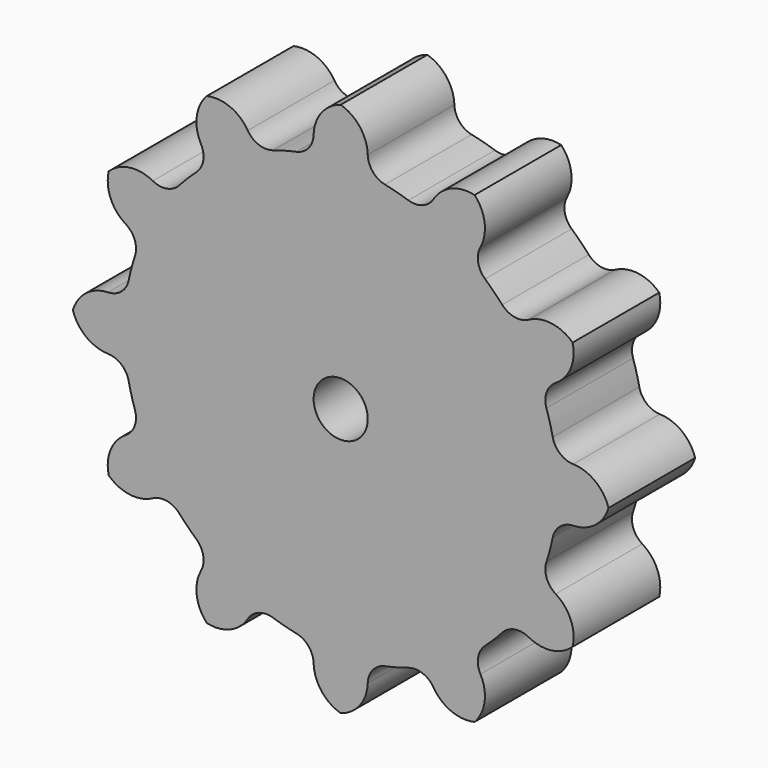
from build123d import *

# Parameters (mm, degrees)
F1_DEPTH    = 25.4
F3_DEPTH    = 25.4
F4_R        = 6.35
F5_DEPTH    = 25.4
F6_T1_DEPTH = 69.85
F7_R        = 5.08


# Not quite as in the source:
# - a fillet or chamfer that OpenCascade refuses, or shapes differently, is made with other operations: its cross-section is extruded or revolved along the edge and cut away or added
# - a feature names something its author has since deleted; it is built from what else it names


with BuildPart() as f1:
    # F0 (on Front) → F1 (new body)
    with BuildSketch(Plane.XZ):
        with BuildLine():
            ThreePointArc((19.7015199239, 46.8240334945), (25.4, 43.9940905122), (30.7000425519, 40.4740334945))
            Line((30.7000425519, 40.4740334945), (37.0901124422, 51.5419592083))
            Line((37.0901124422, 51.5419592083), (26.0915898141, 57.8919592083))
            Line((26.0915898141, 57.8919592083), (19.7015199239, 46.8240334945))
        make_face()
        with BuildLine():
            ThreePointArc((-6.35, 50.4015624758), (0, 50.8), (6.35, 50.4015624758))
            Line((6.35, 50.4015624758), (6.35, 63.1817022563))
            Line((6.35, 63.1817022563), (-6.35, 63.1817022563))
            Line((-6.35, 63.1817022563), (-6.35, 50.4015624758))
        make_face()
        with BuildLine():
            Line((-26.0915898141, -57.8919592083), (-19.7015199239, -46.8240334945))
            ThreePointArc((-19.7015199239, -46.8240334945), (-25.4, -43.9940905122), (-30.7000425519, -40.4740334945))
            Line((-30.7000425519, -40.4740334945), (-37.0901124422, -51.5419592083))
            Line((-37.0901124422, -51.5419592083), (-26.0915898141, -57.8919592083))
        make_face()
        with BuildLine():
            Line((6.35, -63.1817022563), (6.35, -50.4015624758))
            ThreePointArc((6.35, -50.4015624758), (0, -50.8), (-6.35, -50.4015624758))
            Line((-6.35, -50.4015624758), (-6.35, -63.1817022563))
            Line((-6.35, -63.1817022563), (6.35, -63.1817022563))
        make_face()
        with BuildLine():
            Line((30.7000425519, 40.4740334945), (17.3485226281, 17.3485226281))
            Line((17.3485226281, 17.3485226281), (40.4740334945, 30.7000425519))
            ThreePointArc((40.4740334945, 30.7000425519), (35.9210244843, 35.9210244843), (30.7000425519, 40.4740334945))
        make_face()
        with BuildLine():
            Line((6.35, 50.4015624758), (6.35, 23.6985226281))
            Line((6.35, 23.6985226281), (19.7015199239, 46.8240334945))
            ThreePointArc((19.7015199239, 46.8240334945), (13.1480074912, 49.0690319755), (6.35, 50.4015624758))
        make_face()
        with BuildLine():
            Line((-46.8240334945, -19.7015199239), (-6.35, 3.6661742094))
            Line((-6.35, 3.6661742094), (-6.35, 50.4015624758))
            ThreePointArc((-6.35, 50.4015624758), (-43.9940905122, 25.4), (-46.8240334945, -19.7015199239))
        make_face()
        with BuildLine():
            Line((-6.35, -50.4015624758), (-6.35, -23.6985226281))
            Line((-6.35, -23.6985226281), (-19.7015199239, -46.8240334945))
            ThreePointArc((-19.7015199239, -46.8240334945), (-13.1480074912, -49.0690319755), (-6.35, -50.4015624758))
        make_face()
        with BuildLine():
            Line((-30.7000425519, -40.4740334945), (-6.35, 1.7014773719))
            Line((-6.35, 1.7014773719), (-6.35, 3.6661742094))
            Line((-6.35, 3.6661742094), (-46.8240334945, -19.7015199239))
            ThreePointArc((-46.8240334945, -19.7015199239), (-40.1294146696, -31.1491585485), (-30.7000425519, -40.4740334945))
        make_face()
        with BuildLine():
            Line((17.3485226281, 17.3485226281), (6.35, -1.7014773719))
            Line((6.35, -1.7014773719), (6.35, -50.4015624758))
            ThreePointArc((6.35, -50.4015624758), (38.1, -33.6010416505), (50.8, 0))
            ThreePointArc((50.8, 0), (48.149355663, 16.1950470589), (40.4740334945, 30.7000425519))
            Line((40.4740334945, 30.7000425519), (17.3485226281, 17.3485226281))
        make_face()
        with BuildLine():
            Line((6.35, 23.6985226281), (6.35, 10.9985226281))
            Line((6.35, 10.9985226281), (17.3485226281, 17.3485226281))
            Line((17.3485226281, 17.3485226281), (30.7000425519, 40.4740334945))
            ThreePointArc((30.7000425519, 40.4740334945), (25.4, 43.9940905122), (19.7015199239, 46.8240334945))
            Line((19.7015199239, 46.8240334945), (6.35, 23.6985226281))
        make_face()
        with BuildLine():
            Line((-6.35, 3.6661742094), (-4.6485226281, 4.6485226281))
            Line((-4.6485226281, 4.6485226281), (6.35, 23.6985226281))
            Line((6.35, 23.6985226281), (6.35, 50.4015624758))
            ThreePointArc((6.35, 50.4015624758), (0, 50.8), (-6.35, 50.4015624758))
            Line((-6.35, 50.4015624758), (-6.35, 3.6661742094))
        make_face()
        with BuildLine():
            Line((-6.35, -23.6985226281), (-6.35, 1.31e-08))
            Line((-6.35, 1.31e-08), (-6.35, 1.7014773719))
            Line((-6.35, 1.7014773719), (-30.7000425519, -40.4740334945))
            ThreePointArc((-30.7000425519, -40.4740334945), (-25.4, -43.9940905122), (-19.7015199239, -46.8240334945))
            Line((-19.7015199239, -46.8240334945), (-6.35, -23.6985226281))
        make_face()
        with BuildLine():
            Line((6.35, -1.7014773719), (5.4992613469, -3.1749999431))
            Line((5.4992613469, -3.1749999431), (-6.35, -23.6985226281))
            Line((-6.35, -23.6985226281), (-6.35, -50.4015624758))
            ThreePointArc((-6.35, -50.4015624758), (0, -50.8), (6.35, -50.4015624758))
            Line((6.35, -50.4015624758), (6.35, -1.7014773719))
        make_face()
        Polygon((-4.6485226281, 4.6485226281), (-3.1750000958, 5.4992612587), (6.35, 10.9985226281), (6.35, 23.6985226281), align=None)
        with BuildLine():
            ThreePointArc((5.4992613469, -3.1749999431), (6.1336290054, -1.6435009047), (6.35, 0))
            ThreePointArc((6.35, 0), (3.1749999521, 5.4992613417), (-3.1750000958, 5.4992612587))
            ThreePointArc((-3.1750000958, 5.4992612587), (-4.490128147, 4.490127974), (-5.499261381, 3.1749998839))
            ThreePointArc((-5.499261381, 3.1749998839), (-6.1336290126, 1.643500878), (-6.35, 1.31e-08))
            ThreePointArc((-6.35, 1.31e-08), (-1.643500911, -6.1336290037), (5.4992613469, -3.1749999431))
        make_face()
        Polygon((6.35, 10.9985226281), (6.35, 0), (6.35, -1.7014773719), (17.3485226281, 17.3485226281), align=None)
        with BuildLine():
            ThreePointArc((-3.1750000958, 5.4992612587), (3.1749999521, 5.4992613417), (6.35, 0))
            Line((6.35, 0), (6.35, 10.9985226281))
            Line((6.35, 10.9985226281), (-3.1750000958, 5.4992612587))
        make_face()
        with BuildLine():
            Line((-6.35, -23.6985226281), (5.4992613469, -3.1749999431))
            ThreePointArc((5.4992613469, -3.1749999431), (-1.643500911, -6.1336290037), (-6.35, 1.31e-08))
            Line((-6.35, 1.31e-08), (-6.35, -23.6985226281))
        make_face()
        Polygon((-6.35, 1.7014773719), (-5.499261381, 3.1749998839), (-4.6485226281, 4.6485226281), (-6.35, 3.6661742094), align=None)
        with BuildLine():
            Line((6.35, -1.7014773719), (6.35, 0))
            ThreePointArc((6.35, 0), (6.1336290054, -1.6435009047), (5.4992613469, -3.1749999431))
            Line((5.4992613469, -3.1749999431), (6.35, -1.7014773719))
        make_face()
        with BuildLine():
            ThreePointArc((-5.499261381, 3.1749998839), (-4.490128147, 4.490127974), (-3.1750000958, 5.4992612587))
            Line((-3.1750000958, 5.4992612587), (-4.6485226281, 4.6485226281))
            Line((-4.6485226281, 4.6485226281), (-5.499261381, 3.1749998839))
        make_face()
        with BuildLine():
            ThreePointArc((-6.35, 1.31e-08), (-6.1336290126, 1.643500878), (-5.499261381, 3.1749998839))
            Line((-5.499261381, 3.1749998839), (-6.35, 1.7014773719))
            Line((-6.35, 1.7014773719), (-6.35, 1.31e-08))
        make_face()
    extrude(amount=F1_DEPTH)

    # F2 (on Front) → F3 (join)
    with BuildSketch(Plane.XZ):
        with BuildLine():
            ThreePointArc((40.4740334945, 30.7000425519), (43.9940905122, 25.4), (46.8240334945, 19.7015199239))
            Line((46.8240334945, 19.7015199239), (57.8919592083, 26.0915898141))
            Line((57.8919592083, 26.0915898141), (51.5419592083, 37.0901124422))
            Line((51.5419592083, 37.0901124422), (40.4740334945, 30.7000425519))
        make_face()
        with BuildLine():
            ThreePointArc((-30.7000425519, 40.4740334945), (-25.4, 43.9940905122), (-19.7015199239, 46.8240334945))
            Line((-19.7015199239, 46.8240334945), (-26.0915898141, 57.8919592083))
            Line((-26.0915898141, 57.8919592083), (-37.0901124422, 51.5419592083))
            Line((-37.0901124422, 51.5419592083), (-30.7000425519, 40.4740334945))
        make_face()
        with BuildLine():
            ThreePointArc((-46.8240334945, 19.7015199239), (-43.9940905122, 25.4), (-40.4740334945, 30.7000425519))
            Line((-40.4740334945, 30.7000425519), (-51.5419592083, 37.0901124422))
            Line((-51.5419592083, 37.0901124422), (-57.8919592083, 26.0915898141))
            Line((-57.8919592083, 26.0915898141), (-46.8240334945, 19.7015199239))
        make_face()
        with BuildLine():
            Line((-63.1817022563, -6.35), (-50.4015624758, -6.35))
            ThreePointArc((-50.4015624758, -6.35), (-50.8, 0), (-50.4015624758, 6.35))
            Line((-50.4015624758, 6.35), (-63.1817022563, 6.35))
            Line((-63.1817022563, 6.35), (-63.1817022563, -6.35))
        make_face()
        with BuildLine():
            Line((-51.5419592083, -37.0901124422), (-40.4740334945, -30.7000425519))
            ThreePointArc((-40.4740334945, -30.7000425519), (-43.9940905122, -25.4), (-46.8240334945, -19.7015199239))
            Line((-46.8240334945, -19.7015199239), (-57.8919592083, -26.0915898141))
            Line((-57.8919592083, -26.0915898141), (-51.5419592083, -37.0901124422))
        make_face()
        with BuildLine():
            Line((37.0901124422, -51.5419592083), (30.7000425519, -40.4740334945))
            ThreePointArc((30.7000425519, -40.4740334945), (25.4, -43.9940905122), (19.7015199239, -46.8240334945))
            Line((19.7015199239, -46.8240334945), (26.0915898141, -57.8919592083))
            Line((26.0915898141, -57.8919592083), (37.0901124422, -51.5419592083))
        make_face()
        with BuildLine():
            Line((57.8919592083, -26.0915898141), (46.8240334945, -19.7015199239))
            ThreePointArc((46.8240334945, -19.7015199239), (43.9940905122, -25.4), (40.4740334945, -30.7000425519))
            Line((40.4740334945, -30.7000425519), (51.5419592083, -37.0901124422))
            Line((51.5419592083, -37.0901124422), (57.8919592083, -26.0915898141))
        make_face()
        with BuildLine():
            Line((63.1817022563, 6.35), (50.4015624758, 6.35))
            ThreePointArc((50.4015624758, 6.35), (50.7002927692, 3.1812439572), (50.8, 0))
            ThreePointArc((50.8, 0), (50.7002927692, -3.1812439572), (50.4015624758, -6.35))
            Line((50.4015624758, -6.35), (63.1817022563, -6.35))
            Line((63.1817022563, -6.35), (63.1817022563, 6.35))
        make_face()
        with BuildLine():
            Line((46.8240334945, 19.7015199239), (23.6985226281, 6.35))
            Line((23.6985226281, 6.35), (50.4015624758, 6.35))
            ThreePointArc((50.4015624758, 6.35), (49.0690319755, 13.1480074912), (46.8240334945, 19.7015199239))
        make_face()
        with BuildLine():
            Line((-19.7015199239, 46.8240334945), (2.324261314, 8.674261314))
            Line((2.324261314, 8.674261314), (40.4740334945, 30.7000425519))
            ThreePointArc((40.4740334945, 30.7000425519), (13.1480074912, 49.0690319755), (-19.7015199239, 46.8240334945))
        make_face()
        with BuildLine():
            Line((-40.4740334945, 30.7000425519), (-17.3485226281, 17.3485226281))
            Line((-17.3485226281, 17.3485226281), (-30.7000425519, 40.4740334945))
            ThreePointArc((-30.7000425519, 40.4740334945), (-35.9210244843, 35.9210244843), (-40.4740334945, 30.7000425519))
        make_face()
        with BuildLine():
            Line((-50.4015624758, 6.35), (-23.6985226281, 6.35))
            Line((-23.6985226281, 6.35), (-46.8240334945, 19.7015199239))
            ThreePointArc((-46.8240334945, 19.7015199239), (-49.0690319755, 13.1480074912), (-50.4015624758, 6.35))
        make_face()
        with BuildLine():
            Line((-46.8240334945, -19.7015199239), (-23.6985226281, -6.35))
            Line((-23.6985226281, -6.35), (-50.4015624758, -6.35))
            ThreePointArc((-50.4015624758, -6.35), (-49.0690319755, -13.1480074912), (-46.8240334945, -19.7015199239))
        make_face()
        with BuildLine():
            Line((19.7015199239, -46.8240334945), (-2.324261314, -8.674261314))
            Line((-2.324261314, -8.674261314), (-40.4740334945, -30.7000425519))
            ThreePointArc((-40.4740334945, -30.7000425519), (-13.1480074912, -49.0690319755), (19.7015199239, -46.8240334945))
        make_face()
        with BuildLine():
            Line((40.4740334945, -30.7000425519), (17.3485226281, -17.3485226281))
            Line((17.3485226281, -17.3485226281), (30.7000425519, -40.4740334945))
            ThreePointArc((30.7000425519, -40.4740334945), (35.9210244843, -35.9210244843), (40.4740334945, -30.7000425519))
        make_face()
        with BuildLine():
            Line((50.4015624758, -6.35), (23.6985226281, -6.35))
            Line((23.6985226281, -6.35), (46.8240334945, -19.7015199239))
            ThreePointArc((46.8240334945, -19.7015199239), (49.0690319755, -13.1480074912), (50.4015624758, -6.35))
        make_face()
        with BuildLine():
            Line((2.324261314, 8.674261314), (3.6661742094, 6.35))
            Line((3.6661742094, 6.35), (23.6985226281, 6.35))
            Line((23.6985226281, 6.35), (46.8240334945, 19.7015199239))
            ThreePointArc((46.8240334945, 19.7015199239), (43.9940905122, 25.4), (40.4740334945, 30.7000425519))
            Line((40.4740334945, 30.7000425519), (2.324261314, 8.674261314))
        make_face()
        with BuildLine():
            Line((-17.3485226281, 17.3485226281), (0, 7.3323484187))
            Line((0, 7.3323484187), (2.324261314, 8.674261314))
            Line((2.324261314, 8.674261314), (-19.7015199239, 46.8240334945))
            ThreePointArc((-19.7015199239, 46.8240334945), (-25.4, 43.9940905122), (-30.7000425519, 40.4740334945))
            Line((-30.7000425519, 40.4740334945), (-17.3485226281, 17.3485226281))
        make_face()
        with BuildLine():
            Line((-23.6985226281, 6.35), (-10.9985226281, 6.35))
            Line((-10.9985226281, 6.35), (-17.3485226281, 17.3485226281))
            Line((-17.3485226281, 17.3485226281), (-40.4740334945, 30.7000425519))
            ThreePointArc((-40.4740334945, 30.7000425519), (-43.9940905122, 25.4), (-46.8240334945, 19.7015199239))
            Line((-46.8240334945, 19.7015199239), (-23.6985226281, 6.35))
        make_face()
        with BuildLine():
            Line((-23.6985226281, -6.35), (-12.7, 0))
            Line((-12.7, 0), (-23.6985226281, 6.35))
            Line((-23.6985226281, 6.35), (-50.4015624758, 6.35))
            ThreePointArc((-50.4015624758, 6.35), (-50.8, 0), (-50.4015624758, -6.35))
            Line((-50.4015624758, -6.35), (-23.6985226281, -6.35))
        make_face()
        with BuildLine():
            Line((-2.324261314, -8.674261314), (-3.6661742094, -6.35))
            Line((-3.6661742094, -6.35), (-23.6985226281, -6.35))
            Line((-23.6985226281, -6.35), (-46.8240334945, -19.7015199239))
            ThreePointArc((-46.8240334945, -19.7015199239), (-43.9940905122, -25.4), (-40.4740334945, -30.7000425519))
            Line((-40.4740334945, -30.7000425519), (-2.324261314, -8.674261314))
        make_face()
        with BuildLine():
            Line((17.3485226281, -17.3485226281), (0, -7.3323484187))
            Line((0, -7.3323484187), (-2.324261314, -8.674261314))
            Line((-2.324261314, -8.674261314), (19.7015199239, -46.8240334945))
            ThreePointArc((19.7015199239, -46.8240334945), (25.4, -43.9940905122), (30.7000425519, -40.4740334945))
            Line((30.7000425519, -40.4740334945), (17.3485226281, -17.3485226281))
        make_face()
        with BuildLine():
            Line((23.6985226281, -6.35), (10.9985226281, -6.35))
            Line((10.9985226281, -6.35), (17.3485226281, -17.3485226281))
            Line((17.3485226281, -17.3485226281), (40.4740334945, -30.7000425519))
            ThreePointArc((40.4740334945, -30.7000425519), (43.9940905122, -25.4), (46.8240334945, -19.7015199239))
            Line((46.8240334945, -19.7015199239), (23.6985226281, -6.35))
        make_face()
        with BuildLine():
            Line((23.6985226281, 6.35), (12.7, 0))
            Line((12.7, 0), (23.6985226281, -6.35))
            Line((23.6985226281, -6.35), (50.4015624758, -6.35))
            ThreePointArc((50.4015624758, -6.35), (50.7002927692, -3.1812439572), (50.8, 0))
            ThreePointArc((50.8, 0), (50.7002927692, 3.1812439572), (50.4015624758, 6.35))
            Line((50.4015624758, 6.35), (23.6985226281, 6.35))
        make_face()
        Polygon((-12.7, 0), (-8.674261314, 2.324261314), (-10.9985226281, 6.35), (-23.6985226281, 6.35), align=None)
        with BuildLine():
            ThreePointArc((-5.4992614049, -3.1749998425), (-6.1336289764, 1.643501013), (-3.1750000201, 5.4992613024))
            Line((-3.1750000201, 5.4992613024), (-8.674261314, 2.324261314))
            Line((-8.674261314, 2.324261314), (-5.4992614049, -3.1749998425))
        make_face()
        Polygon((3.6661742094, 6.35), (4.6485226281, 4.6485226281), (12.7, 0), (23.6985226281, 6.35), align=None)
        Polygon((8.674261314, -2.324261314), (3.1750001359, -5.4992612355), (1.7014773719, -6.35), (10.9985226281, -6.35), align=None)
        Polygon((-3.6661742094, -6.35), (-4.6485226281, -4.6485226281), (-12.7, 0), (-23.6985226281, -6.35), align=None)
        Polygon((-10.9985226281, 6.35), (-1.7014773719, 6.35), (0, 7.3323484187), (-17.3485226281, 17.3485226281), align=None)
        Polygon((-4.6485226281, -4.6485226281), (-5.4992614049, -3.1749998425), (-8.674261314, 2.324261314), (-12.7, 0), align=None)
        Polygon((10.9985226281, -6.35), (1.7014773719, -6.35), (0, -7.3323484187), (17.3485226281, -17.3485226281), align=None)
        Polygon((4.6485226281, 4.6485226281), (5.4992613044, 3.1750000167), (8.674261314, -2.324261314), (12.7, 0), align=None)
        Polygon((0, -7.3323484187), (-1.7014773719, -6.35), (-3.6661742094, -6.35), (-2.324261314, -8.674261314), align=None)
        with BuildLine():
            ThreePointArc((5.4992613044, 3.1750000167), (6.1336289944, 1.6435009457), (6.35, 0))
            ThreePointArc((6.35, 0), (5.4992613533, -3.174999932), (3.1750001359, -5.4992612355))
            Line((3.1750001359, -5.4992612355), (8.674261314, -2.324261314))
            Line((8.674261314, -2.324261314), (5.4992613044, 3.1750000167))
        make_face()
        Polygon((-8.674261314, 2.324261314), (-3.1750000201, 5.4992613024), (-1.7014773719, 6.35), (-10.9985226281, 6.35), align=None)
        Polygon((12.7, 0), (8.674261314, -2.324261314), (10.9985226281, -6.35), (23.6985226281, -6.35), align=None)
        Polygon((1.7014773719, -6.35), (3.51e-08, -6.35), (-1.7014773719, -6.35), (0, -7.3323484187), align=None)
        Polygon((1.7014773719, 6.35), (3.1750001989, 5.4992611992), (4.6485226281, 4.6485226281), (3.6661742094, 6.35), align=None)
        Polygon((0, 7.3323484187), (1.7014773719, 6.35), (3.6661742094, 6.35), (2.324261314, 8.674261314), align=None)
        Polygon((-1.7014773719, -6.35), (-3.174999941, -5.4992613481), (-4.6485226281, -4.6485226281), (-3.6661742094, -6.35), align=None)
        with BuildLine():
            ThreePointArc((3.1750001359, -5.4992612355), (5.4992613533, -3.174999932), (6.35, 0))
            ThreePointArc((6.35, 0), (6.1336289944, 1.6435009457), (5.4992613044, 3.1750000167))
            ThreePointArc((5.4992613044, 3.1750000167), (4.4901281349, 4.4901279862), (3.1750001989, 5.4992611992))
            ThreePointArc((3.1750001989, 5.4992611992), (1.6435010473, 6.1336289672), (0, 6.35))
            ThreePointArc((0, 6.35), (-1.6435009476, 6.1336289939), (-3.1750000201, 5.4992613024))
            ThreePointArc((-3.1750000201, 5.4992613024), (-6.1336289764, 1.643501013), (-5.4992614049, -3.1749998425))
            ThreePointArc((-5.4992614049, -3.1749998425), (-4.4901281007, -4.4901280203), (-3.174999941, -5.4992613481))
            ThreePointArc((-3.174999941, -5.4992613481), (-1.6435008865, -6.1336290103), (3.51e-08, -6.35))
            ThreePointArc((3.51e-08, -6.35), (1.6435010292, -6.1336289721), (3.1750001359, -5.4992612355))
        make_face()
        with BuildLine():
            ThreePointArc((-3.1750000201, 5.4992613024), (-1.6435009476, 6.1336289939), (0, 6.35))
            Line((0, 6.35), (-1.7014773719, 6.35))
            Line((-1.7014773719, 6.35), (-3.1750000201, 5.4992613024))
        make_face()
        with BuildLine():
            Line((1.7014773719, -6.35), (3.1750001359, -5.4992612355))
            ThreePointArc((3.1750001359, -5.4992612355), (1.6435010292, -6.1336289721), (3.51e-08, -6.35))
            Line((3.51e-08, -6.35), (1.7014773719, -6.35))
        make_face()
        Polygon((-1.7014773719, 6.35), (0, 6.35), (1.7014773719, 6.35), (0, 7.3323484187), align=None)
        with BuildLine():
            ThreePointArc((0, 6.35), (1.6435010473, 6.1336289672), (3.1750001989, 5.4992611992))
            Line((3.1750001989, 5.4992611992), (1.7014773719, 6.35))
            Line((1.7014773719, 6.35), (0, 6.35))
        make_face()
        with BuildLine():
            Line((-1.7014773719, -6.35), (3.51e-08, -6.35))
            ThreePointArc((3.51e-08, -6.35), (-1.6435008865, -6.1336290103), (-3.174999941, -5.4992613481))
            Line((-3.174999941, -5.4992613481), (-1.7014773719, -6.35))
        make_face()
        with BuildLine():
            Line((-4.6485226281, -4.6485226281), (-3.174999941, -5.4992613481))
            ThreePointArc((-3.174999941, -5.4992613481), (-4.4901281007, -4.4901280203), (-5.4992614049, -3.1749998425))
            Line((-5.4992614049, -3.1749998425), (-4.6485226281, -4.6485226281))
        make_face()
        with BuildLine():
            ThreePointArc((3.1750001989, 5.4992611992), (4.4901281349, 4.4901279862), (5.4992613044, 3.1750000167))
            Line((5.4992613044, 3.1750000167), (4.6485226281, 4.6485226281))
            Line((4.6485226281, 4.6485226281), (3.1750001989, 5.4992611992))
        make_face()
    extrude(amount=F3_DEPTH)

    # F4 (on face) → F5 (cut)
    with BuildSketch(Plane.XZ.offset(25.4)):
        Circle(F4_R)
    extrude(amount=-F5_DEPTH, mode=Mode.SUBTRACT)

    # F6: fillet of radius 8.89 on 24 edges, made by hand

    # F6_s2 → F6_t1 (cut)
    with BuildSketch(Plane.XZ.offset(-22.225)):
        with BuildLine():
            ThreePointArc((2.54, 63.1817022563), (-3.7461792847, 60.577881541), (-6.35, 54.2917022563))
            Line((-6.35, 54.2917022563), (-6.35, 63.1817022563))
            Line((-6.35, 63.1817022563), (2.54, 63.1817022563))
        make_face()
        with BuildLine():
            ThreePointArc((6.35, 54.2917022563), (3.7461792847, 60.577881541), (-2.54, 63.1817022563))
            Line((-2.54, 63.1817022563), (6.35, 63.1817022563))
            Line((6.35, 63.1817022563), (6.35, 54.2917022563))
        make_face()
        with BuildLine():
            ThreePointArc((33.7905556537, 53.4469592083), (27.0446543428, 54.3350739643), (21.6465898141, 50.1929933686))
            Line((21.6465898141, 50.1929933686), (26.0915898141, 57.8919592083))
            Line((26.0915898141, 57.8919592083), (33.7905556537, 53.4469592083))
        make_face()
        with BuildLine():
            ThreePointArc((32.6451124422, 43.8429933686), (33.5332271982, 50.5888946796), (29.3911466025, 55.9869592083))
            Line((29.3911466025, 55.9869592083), (37.0901124422, 51.5419592083))
            Line((37.0901124422, 51.5419592083), (32.6451124422, 43.8429933686))
        make_face()
        with BuildLine():
            ThreePointArc((43.8429933686, 32.6451124422), (50.5888946796, 33.5332271982), (55.9869592083, 29.3911466025))
            Line((55.9869592083, 29.3911466025), (51.5419592083, 37.0901124422))
            Line((51.5419592083, 37.0901124422), (43.8429933686, 32.6451124422))
        make_face()
        with BuildLine():
            ThreePointArc((53.4469592083, 33.7905556537), (54.3350739643, 27.0446543428), (50.1929933686, 21.6465898141))
            Line((50.1929933686, 21.6465898141), (57.8919592083, 26.0915898141))
            Line((57.8919592083, 26.0915898141), (53.4469592083, 33.7905556537))
        make_face()
        with BuildLine():
            ThreePointArc((-21.6465898141, 50.1929933686), (-27.0446543428, 54.3350739643), (-33.7905556537, 53.4469592083))
            Line((-33.7905556537, 53.4469592083), (-26.0915898141, 57.8919592083))
            Line((-26.0915898141, 57.8919592083), (-21.6465898141, 50.1929933686))
        make_face()
        with BuildLine():
            ThreePointArc((-29.3911466025, 55.9869592083), (-33.5332271982, 50.5888946796), (-32.6451124422, 43.8429933686))
            Line((-32.6451124422, 43.8429933686), (-37.0901124422, 51.5419592083))
            Line((-37.0901124422, 51.5419592083), (-29.3911466025, 55.9869592083))
        make_face()
        with BuildLine():
            ThreePointArc((-43.8429933686, 32.6451124422), (-50.5888946796, 33.5332271982), (-55.9869592083, 29.3911466025))
            Line((-55.9869592083, 29.3911466025), (-51.5419592083, 37.0901124422))
            Line((-51.5419592083, 37.0901124422), (-43.8429933686, 32.6451124422))
        make_face()
        with BuildLine():
            ThreePointArc((-53.4469592083, 33.7905556537), (-54.3350739643, 27.0446543428), (-50.1929933686, 21.6465898141))
            Line((-50.1929933686, 21.6465898141), (-57.8919592083, 26.0915898141))
            Line((-57.8919592083, 26.0915898141), (-53.4469592083, 33.7905556537))
        make_face()
        with BuildLine():
            ThreePointArc((-54.2917022563, 6.35), (-60.577881541, 3.7461792847), (-63.1817022563, -2.54))
            Line((-63.1817022563, -2.54), (-63.1817022563, 6.35))
            Line((-63.1817022563, 6.35), (-54.2917022563, 6.35))
        make_face()
        with BuildLine():
            ThreePointArc((-63.1817022563, 2.54), (-60.577881541, -3.7461792847), (-54.2917022563, -6.35))
            Line((-54.2917022563, -6.35), (-63.1817022563, -6.35))
            Line((-63.1817022563, -6.35), (-63.1817022563, 2.54))
        make_face()
        with BuildLine():
            ThreePointArc((-55.9869592083, -29.3911466025), (-50.5888946796, -33.5332271982), (-43.8429933686, -32.6451124422))
            Line((-43.8429933686, -32.6451124422), (-51.5419592083, -37.0901124422))
            Line((-51.5419592083, -37.0901124422), (-55.9869592083, -29.3911466025))
        make_face()
        with BuildLine():
            ThreePointArc((-50.1929933686, -21.6465898141), (-54.3350739643, -27.0446543428), (-53.4469592083, -33.7905556537))
            Line((-53.4469592083, -33.7905556537), (-57.8919592083, -26.0915898141))
            Line((-57.8919592083, -26.0915898141), (-50.1929933686, -21.6465898141))
        make_face()
        with BuildLine():
            ThreePointArc((-32.6451124422, -43.8429933686), (-33.5332271982, -50.5888946796), (-29.3911466025, -55.9869592083))
            Line((-29.3911466025, -55.9869592083), (-37.0901124422, -51.5419592083))
            Line((-37.0901124422, -51.5419592083), (-32.6451124422, -43.8429933686))
        make_face()
        with BuildLine():
            ThreePointArc((-33.7905556537, -53.4469592083), (-27.0446543428, -54.3350739643), (-21.6465898141, -50.1929933686))
            Line((-21.6465898141, -50.1929933686), (-26.0915898141, -57.8919592083))
            Line((-26.0915898141, -57.8919592083), (-33.7905556537, -53.4469592083))
        make_face()
        with BuildLine():
            ThreePointArc((2.54, -63.1817022563), (-3.7461792847, -60.577881541), (-6.35, -54.2917022563))
            Line((-6.35, -54.2917022563), (-6.35, -63.1817022563))
            Line((-6.35, -63.1817022563), (2.54, -63.1817022563))
        make_face()
        with BuildLine():
            ThreePointArc((6.35, -54.2917022563), (3.7461792847, -60.577881541), (-2.54, -63.1817022563))
            Line((-2.54, -63.1817022563), (6.35, -63.1817022563))
            Line((6.35, -63.1817022563), (6.35, -54.2917022563))
        make_face()
        with BuildLine():
            ThreePointArc((33.7905556537, -53.4469592083), (27.0446543428, -54.3350739643), (21.6465898141, -50.1929933686))
            Line((21.6465898141, -50.1929933686), (26.0915898141, -57.8919592083))
            Line((26.0915898141, -57.8919592083), (33.7905556537, -53.4469592083))
        make_face()
        with BuildLine():
            ThreePointArc((32.6451124422, -43.8429933686), (33.5332271982, -50.5888946796), (29.3911466025, -55.9869592083))
            Line((29.3911466025, -55.9869592083), (37.0901124422, -51.5419592083))
            Line((37.0901124422, -51.5419592083), (32.6451124422, -43.8429933686))
        make_face()
        with BuildLine():
            ThreePointArc((55.9869592083, -29.3911466025), (50.5888946796, -33.5332271982), (43.8429933686, -32.6451124422))
            Line((43.8429933686, -32.6451124422), (51.5419592083, -37.0901124422))
            Line((51.5419592083, -37.0901124422), (55.9869592083, -29.3911466025))
        make_face()
        with BuildLine():
            ThreePointArc((50.1929933686, -21.6465898141), (54.3350739643, -27.0446543428), (53.4469592083, -33.7905556537))
            Line((53.4469592083, -33.7905556537), (57.8919592083, -26.0915898141))
            Line((57.8919592083, -26.0915898141), (50.1929933686, -21.6465898141))
        make_face()
        with BuildLine():
            ThreePointArc((63.1817022563, 2.54), (60.577881541, -3.7461792847), (54.2917022563, -6.35))
            Line((54.2917022563, -6.35), (63.1817022563, -6.35))
            Line((63.1817022563, -6.35), (63.1817022563, 2.54))
        make_face()
        with BuildLine():
            ThreePointArc((54.2917022563, 6.35), (60.577881541, 3.7461792847), (63.1817022563, -2.54))
            Line((63.1817022563, -2.54), (63.1817022563, 6.35))
            Line((63.1817022563, 6.35), (54.2917022563, 6.35))
        make_face()
    extrude(amount=F6_T1_DEPTH, mode=Mode.SUBTRACT)

    # F7
    f7_edges = [f1.edges().sort_by_distance(p)[0] for p in [
        (-19.70152, -12.7, 46.824033),
        (-6.35, -12.7, 50.401562),
        (-40.474033, -12.7, 30.700043),
        (-30.700043, -12.7, 40.474033),
        (-50.401562, -12.7, 6.35),
        (-46.824033, -12.7, 19.70152),
        (-46.824033, -12.7, -19.70152),
        (-50.401562, -12.7, -6.35),
        (-40.474033, -12.7, -30.700043),
        (-30.700043, -12.7, -40.474033),
        (-19.70152, -12.7, -46.824033),
        (-6.35, -12.7, -50.401562),
        (6.35, -12.7, -50.401562),
        (19.70152, -12.7, -46.824033),
        (40.474033, -12.7, -30.700043),
        (30.700043, -12.7, -40.474033),
        (50.401562, -12.7, -6.35),
        (46.824033, -12.7, -19.70152),
        (50.401562, -12.7, 6.35),
        (46.824033, -12.7, 19.70152),
        (40.474033, -12.7, 30.700043),
        (30.700043, -12.7, 40.474033),
        (6.35, -12.7, 50.401562),
        (19.70152, -12.7, 46.824033),
    ]]
    fillet(f7_edges, radius=F7_R)


solid = f1.part
